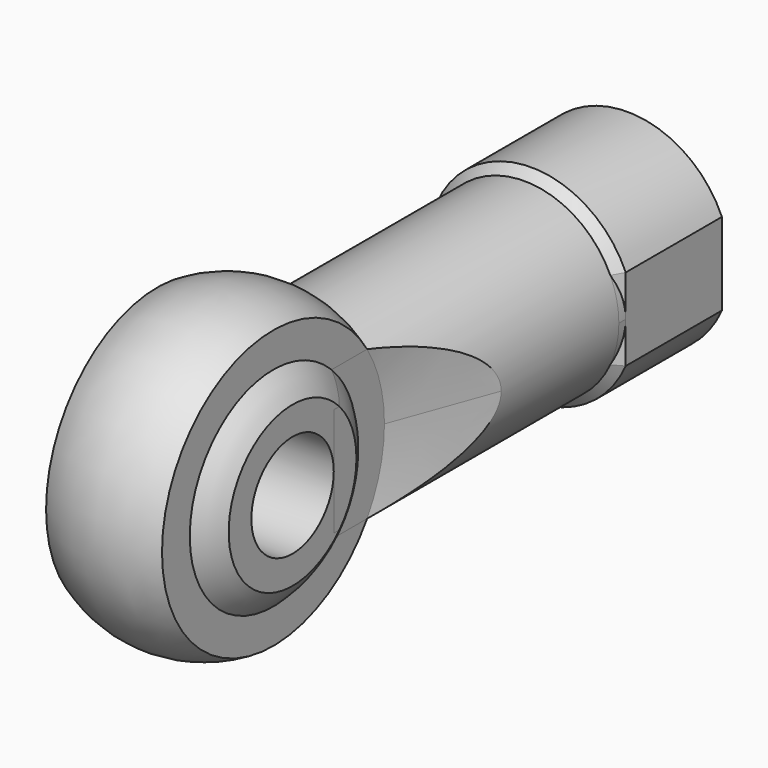
from build123d import *

# Parameters (mm, degrees)
F9_R          = 3
F10_DEPTH     = 27
F11_DEPTH     = 7.5
F12_DEPTH     = 13.5
F13_T2_ANGLE  = 157.4663491
F13_T6_DEPTH  = 3.6837572556
F13_S7_R      = 5.5
F13_T8_DEPTH  = 3
F13_T12_DEPTH = 3.6837572556
F13_S13_R     = 5.5
F13_T14_DEPTH = 3
F13_T16_ANGLE = 157.4663491
F13_T20_DEPTH = 3.6837572556
F13_S21_R     = 5.5
F13_T22_DEPTH = 3
F13_T26_DEPTH = 3.6837572556
F13_S27_R     = 5.5
F13_T28_DEPTH = 3


# Not quite as in the source:
# - a fillet or chamfer that OpenCascade refuses, or shapes differently, is made with other operations: its cross-section is extruded or revolved along the edge and cut away or added


with BuildPart() as f7:
    # F6 (on Top) → F7 (revolve)
    with BuildSketch(Plane.XY):
        with BuildLine():
            Line((-4.5, 4.65), (-4.5, 3))
            Line((-4.5, 3), (4.5, 3))
            Line((4.5, 3), (4.5, 4.65))
            ThreePointArc((4.5, 4.65), (4.0013141648, 5.4121962233), (3.375, 6.073529129))
            ThreePointArc((3.375, 6.073529129), (0, 7.35), (-3.375, 6.073529129))
            ThreePointArc((-3.375, 6.073529129), (-4.0013141648, 5.4121962233), (-4.5, 4.65))
        make_face()
        with BuildLine():
            Line((-3.375, 8.0956714755), (-3.375, 6.073529129))
            ThreePointArc((-3.375, 6.073529129), (0, 7.35), (3.375, 6.073529129))
            Line((3.375, 6.073529129), (3.375, 8.0956714755))
            ThreePointArc((3.375, 8.0956714755), (0, 9), (-3.375, 8.0956714755))
        make_face()
    revolve(axis=Axis((0, 0, 0), (1, 0, 0)))

    # F9 (on offset) → F10 (join)
    with BuildSketch(Plane.XZ.offset(-30)):
        with BuildLine():
            ThreePointArc((-5.5, 0), (0, -5.5), (5.5, 0))
            ThreePointArc((5.5, 0), (0, 5.5), (-5.5, 0))
        make_face()
        Circle(F9_R, mode=Mode.SUBTRACT)
        Circle(F9_R)
    extrude(amount=F10_DEPTH)

    # F9 (on offset) → F11 (join)
    with BuildSketch(Plane.XZ.offset(-30)):
        with BuildLine():
            ThreePointArc((-5.5, 0), (0, 5.5), (5.5, 0))
            Line((5.5, 0), (5.5, 2.3979157617))
            ThreePointArc((5.5, 2.3979157617), (0, 6), (-5.5, 2.3979157617))
            Line((-5.5, 2.3979157617), (-5.5, 0))
        make_face()
        with BuildLine():
            Line((5.5, -2.3979157617), (5.5, 0))
            ThreePointArc((5.5, 0), (0, -5.5), (-5.5, 0))
            Line((-5.5, 0), (-5.5, -2.3979157617))
            ThreePointArc((-5.5, -2.3979157617), (0, -6), (5.5, -2.3979157617))
        make_face()
    extrude(amount=F11_DEPTH)

    # F9 (on offset) → F12 (cut)
    with BuildSketch(Plane.XZ.offset(-30)):
        Circle(F9_R)
    extrude(amount=F12_DEPTH, mode=Mode.SUBTRACT)

    # F13: chamfer of 0.5 on 6 edges, made by hand

    # F13_s1 → F13_t2 (revolve, cut)
    with BuildSketch(Plane(origin=(0, 0, 0), x_dir=(0, 1, 0), z_dir=(0.1953783305, 0, -0.980727948))):
        Polygon((22.5, 5.5), (23, 6), (22.5, 6), align=None)
    revolve(axis=Axis((0, 22.5, 0), (0, -1, 0)), revolution_arc=F13_T2_ANGLE, mode=Mode.SUBTRACT)


with BuildPart() as f13_tool4:
    # F13_s5 → F13_t6 (new body)
    with BuildSketch(Plane.XY):
        Polygon((5, 22.5), (5.5, 23), (5.5, 22.5), align=None)
    extrude(amount=F13_T6_DEPTH)

    # F13_s7 → F13_t8 (cut, symmetric)
    with BuildSketch(Plane.XZ.offset(-22.8)):
        Circle(F13_S7_R)
    extrude(amount=F13_T8_DEPTH, both=True, mode=Mode.SUBTRACT)


with BuildPart() as f7_1:
    add(f7.part)

    # F13_t3: cut F13_tool4
    add(f13_tool4.part, mode=Mode.SUBTRACT)


with BuildPart() as f13_tool10:
    # F13_s11 → F13_t12 (new body)
    with BuildSketch(Plane.XY.offset(3.6837572556)):
        Polygon((-5, 22.5), (-5.5, 23), (-5.5, 22.5), align=None)
    extrude(amount=-F13_T12_DEPTH)

    # F13_s13 → F13_t14 (cut, symmetric)
    with BuildSketch(Plane.XZ.offset(-22.8)):
        Circle(F13_S13_R)
    extrude(amount=F13_T14_DEPTH, both=True, mode=Mode.SUBTRACT)


with BuildPart() as f7_2:
    add(f7_1.part)

    # F13_t9: cut F13_tool10
    add(f13_tool10.part, mode=Mode.SUBTRACT)

    # F13_s15 → F13_t16 (revolve, cut)
    with BuildSketch(Plane(origin=(0, 0, 0), x_dir=(0, 1, 0), z_dir=(-0.1953783305, 0, 0.980727948))):
        Polygon((22.5, 5.5), (23, 6), (22.5, 6), align=None)
    revolve(axis=Axis((0, 22.5, 0), (0, -1, 0)), revolution_arc=F13_T16_ANGLE, mode=Mode.SUBTRACT)


with BuildPart() as f13_tool18:
    # F13_s19 → F13_t20 (new body)
    with BuildSketch(Plane.XY.offset(-3.6837572556)):
        Polygon((5, 22.5), (5.5, 23), (5.5, 22.5), align=None)
    extrude(amount=F13_T20_DEPTH)

    # F13_s21 → F13_t22 (cut, symmetric)
    with BuildSketch(Plane.XZ.offset(-22.8)):
        Circle(F13_S21_R)
    extrude(amount=F13_T22_DEPTH, both=True, mode=Mode.SUBTRACT)


with BuildPart() as f7_3:
    add(f7_2.part)

    # F13_t17: cut F13_tool18
    add(f13_tool18.part, mode=Mode.SUBTRACT)


with BuildPart() as f13_tool24:
    # F13_s25 → F13_t26 (new body)
    with BuildSketch(Plane.XY):
        Polygon((-5, 22.5), (-5.5, 23), (-5.5, 22.5), align=None)
    extrude(amount=-F13_T26_DEPTH)

    # F13_s27 → F13_t28 (cut, symmetric)
    with BuildSketch(Plane.XZ.offset(-22.8)):
        Circle(F13_S27_R)
    extrude(amount=F13_T28_DEPTH, both=True, mode=Mode.SUBTRACT)


with BuildPart() as f7_4:
    add(f7_3.part)

    # F13_t23: cut F13_tool24
    add(f13_tool24.part, mode=Mode.SUBTRACT)

    # F6 (on Top) → F14 (revolve, cut)
    with BuildSketch(Plane.XY):
        with BuildLine():
            Line((4.5, 4.65), (4.5, 3))
            Line((4.5, 3), (6.5, 3))
            Line((6.5, 3), (6.5, 16.6815384113))
            Line((6.5, 16.6815384113), (3.375, 8.0956714755))
            Line((3.375, 8.0956714755), (3.375, 6.073529129))
            ThreePointArc((3.375, 6.073529129), (4.0013141648, 5.4121962233), (4.5, 4.65))
        make_face()
        with BuildLine():
            Line((-6.5, 3), (-4.5, 3))
            Line((-4.5, 3), (-4.5, 4.65))
            ThreePointArc((-4.5, 4.65), (-4.0013141648, 5.4121962233), (-3.375, 6.073529129))
            Line((-3.375, 6.073529129), (-3.375, 8.0956714755))
            Line((-3.375, 8.0956714755), (-6.5, 16.6815384113))
            Line((-6.5, 16.6815384113), (-6.5, 3))
        make_face()
    revolve(axis=Axis((0, 0, 0), (1, 0, 0)), mode=Mode.SUBTRACT)


solid = f7_4.part
